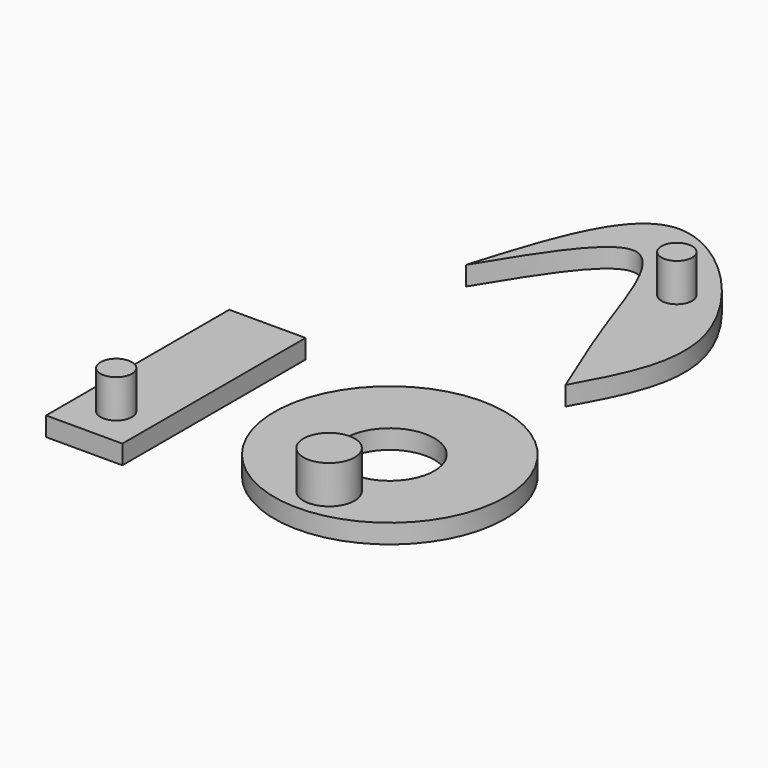
from build123d import *

# Parameters (mm, degrees)
F0_W     = 25.4
F0_H     = 76.2
F1_DEPTH = 6.35
F0_R     = 38.4394579133
F0_R_2   = 14.8046934969
F2_R     = 5.2316610028
F3_DEPTH = 12.7
F2_R_2   = 8.5125938891
F2_R_3   = 5.1188797051


with BuildPart() as f1:
    # F0 (on Top) → F1 (new body)
    with BuildSketch(Plane.XY):
        with Locations((-49.2798545945, -0.5338639021)):
            Rectangle(F0_W, F0_H)
    extrude(amount=F1_DEPTH)

    # F2 (on face) → F3 (join)
    with BuildSketch(Plane.XY.offset(6.35)):
        with Locations((-49.2086187005, -25.410592556)):
            Circle(F2_R)
    extrude(amount=F3_DEPTH)


with BuildPart() as f1b:
    # F0 (on Top) → F1, piece 2 (new body)
    with BuildSketch(Plane.XY):
        with Locations((21.5263813734, 0)):
            Circle(F0_R)
        with Locations((21.5263813734, 0)):
            Circle(F0_R_2, mode=Mode.SUBTRACT)
    extrude(amount=F1_DEPTH)

    # F2 (on face) → F3, piece 2 (join)
    with BuildSketch(Plane.XY.offset(6.35)):
        with Locations((22.1362113953, -26.0249078274)):
            Circle(F2_R_2)
    extrude(amount=F3_DEPTH)


with BuildPart() as f1c:
    # F0 (on Top) → F1, piece 3 (new body)
    with BuildSketch(Plane.XY):
        with BuildLine():
            add(Edge.make_bspline(
                [(-29.7179743648, 95.7142338157), (-19.0131454807, 113.233737551), (1.5796451251, 146.9358558674), (19.0124895635, 92.0655705958), (28.123248858, 70.1702824146), (32.7103585005, 59.1463893652)],
                knots=[0, 0, 0, 0, 0.3496087633, 0.6725394057, 1, 1, 1, 1], degree=3))
            add(Edge.make_bspline(
                [(32.7103585005, 59.1463893652), (40.5245970676, 73.2035069742), (57.2342930122, 103.2627499743), (-7.2032755891, 170.1391956814), (-22.2476159218, 120.4084125144), (-29.7179743648, 95.7142338157)],
                knots=[0, 0, 0, 0, 0.3066393633, 0.6557067286, 1, 1, 1, 1], degree=3))
        make_face()
    extrude(amount=F1_DEPTH)

    # F2 (on face) → F3, piece 3 (join)
    with BuildSketch(Plane.XY.offset(6.35)):
        with Locations((23.7596780062, 116.629704833)):
            Circle(F2_R_3)
    extrude(amount=F3_DEPTH)


solid = Compound([f1.part, f1b.part, f1c.part])
